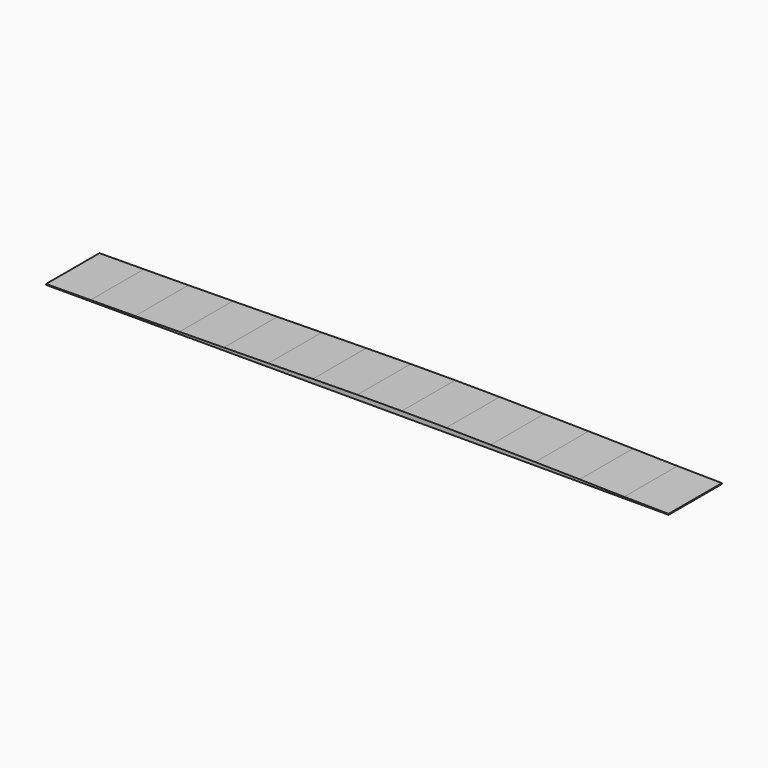
from build123d import *

# Parameters (mm, degrees)
F1_DEPTH = 150


# Not quite as in the source:
# - ends of sketch curves that miss each other by under 0.0002 mm in the source are joined


with BuildPart() as f1:
    # F0 (on Front) → F1 (new body)
    with BuildSketch(Plane.XZ):
        Polygon((-699.999977, -3.250003), (-699.999977, -5.250003), (700, -5.249997), (700, -3.249997), (600, -1.999997), (500, 3e-06), (400, 1.850003), (300, 3.400003), (200, 4.650003), (100, 5.250003), (0, 4.950003), (-100, 3.750003), (-200, 2.250003), (-300, 0.800003), (-400, -0.499997), (-500, -1.699997), (-600, -2.549997), align=None)
    extrude(amount=F1_DEPTH)


solid = f1.part
